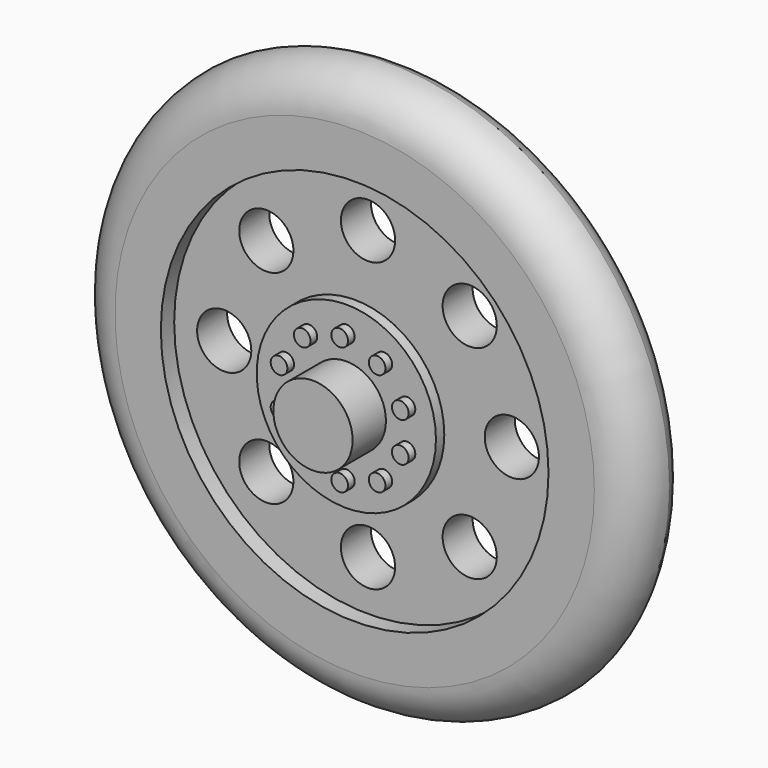
from build123d import *

# Parameters (mm, degrees)
F0_R      = 17.145
F1_DEPTH  = 4.318
F2_R      = 2.54
F4_R      = 5.461
F5_DEPTH  = 0.635
F6_R      = 2.413
F7_DEPTH  = 2.54
F9_R      = 1.651
F10_DEPTH = 25.4
F11_R     = 0.508
F12_DEPTH = 0.508
F8_R      = 11.811
F13_DEPTH = 1.016
F14_R     = 11.811
F15_DEPTH = 1.016
F16_R     = 1.524
F17_DEPTH = 5.08


# Not quite as in the source:
# - a fillet or chamfer that OpenCascade refuses, or shapes differently, is made with other operations: its cross-section is extruded or revolved along the edge and cut away or added


with BuildPart() as f1:
    # F0 (on Front) → F1 (new body)
    with BuildSketch(Plane.XZ):
        Circle(F0_R)
    extrude(amount=-F1_DEPTH)

    # F2
    f2_edges = [f1.edges().sort_by_distance(p)[0] for p in [
        (-17.145, 0, 0),
    ]]
    fillet(f2_edges, radius=F2_R)

    # F3: fillet of radius 2.54 on 1 edges, made by hand

    # F3_s1 → F3_t2 (revolve, cut)
    with BuildSketch(Plane.XY):
        with BuildLine():
            ThreePointArc((17.145, 2.54), (16.2246786933, 3.8258134681), (14.7219944284, 4.318))
            Line((14.7219944284, 4.318), (17.145, 4.318))
            Line((17.145, 4.318), (17.145, 2.54))
        make_face()
    revolve(axis=Axis((0, 4.318, 0), (0, -1, 0)), mode=Mode.SUBTRACT)

    # F9 (on face) → F10 (cut)
    with BuildSketch(Plane.XZ):
        with Locations((0, -8.7630003691)):
            Circle(F9_R)
        with Locations((6.1963769845, -6.1963769845)):
            Circle(F9_R)
        with Locations((8.7630003691, 0)):
            Circle(F9_R)
        with Locations((6.1963769845, 6.1963769845)):
            Circle(F9_R)
        with Locations((-8.7630003691, 0)):
            Circle(F9_R)
        with Locations((0, 8.7630003691)):
            Circle(F9_R)
        with Locations((-6.1963769845, 6.1963769845)):
            Circle(F9_R)
        with Locations((-6.1963769845, -6.1963769845)):
            Circle(F9_R)
    extrude(amount=-F10_DEPTH, mode=Mode.SUBTRACT)

    # F8 (on face) → F13 (cut)
    with BuildSketch(Plane.XZ):
        Circle(F8_R)
    extrude(amount=-F13_DEPTH, mode=Mode.SUBTRACT)

    # F14 (on face) → F15 (cut)
    with BuildSketch(Plane(origin=(0, 4.318, 0), x_dir=(-1, 0, 0), z_dir=(0, 1, 0))):
        Circle(F14_R)
    extrude(amount=-F15_DEPTH, mode=Mode.SUBTRACT)

    # F16 (on face) → F17 (join)
    with BuildSketch(Plane(origin=(0, 3.302, 0), x_dir=(-1, 0, 0), z_dir=(0, 1, 0))):
        Circle(F16_R)
    extrude(amount=F17_DEPTH)


with BuildPart() as f5:
    # F4 (on face) → F5 (new body)
    with BuildSketch(Plane.XZ):
        Circle(F4_R)
    extrude(amount=F5_DEPTH)

    # F6 (on face) → F7 (join)
    with BuildSketch(Plane.XZ.offset(0.635)):
        Circle(F6_R)
    extrude(amount=F7_DEPTH)

    # F11 (on face) → F12 (join)
    with BuildSketch(Plane.XZ.offset(0.635)):
        with Locations((0, 3.8840922061)):
            Circle(F11_R)
        with Locations((-2.2830121173, 3.1422966025)):
            Circle(F11_R)
        with Locations((-3.6939912025, 1.2002504994)):
            Circle(F11_R)
        with Locations((-3.6939912025, -1.2002504994)):
            Circle(F11_R)
        with Locations((-2.2830121173, -3.1422966025)):
            Circle(F11_R)
        with Locations((0, -3.8840922061)):
            Circle(F11_R)
        with Locations((2.2830121173, 3.1422966025)):
            Circle(F11_R)
        with Locations((3.6939912025, 1.2002504994)):
            Circle(F11_R)
        with Locations((3.6939912025, -1.2002504994)):
            Circle(F11_R)
        with Locations((2.2830121173, -3.1422966025)):
            Circle(F11_R)
    extrude(amount=F12_DEPTH)


solid = Compound([f1.part, f5.part])
